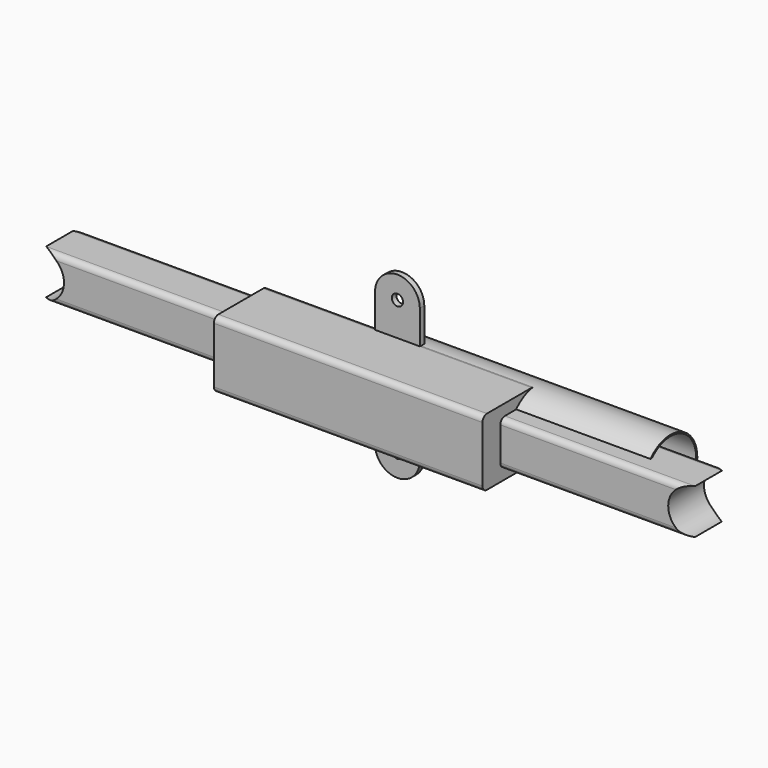
from build123d import *

# Parameters (mm, degrees)
F1_DEPTH    = 50.8
F2_R        = 6.35
F3_R        = 25.4
F3_R_2      = 22.225
F4_DEPTH    = 50.8
F6_DEPTH    = 50.8
F7_T1_DEPTH = 990.6
F8_R        = 6.35
F9_DEPTH    = 6.35
F10_R       = 22.225
F10_R_2     = 6.35
F11_DEPTH   = 50.8
F12_R       = 25.4
F12_R_2     = 6.35
F13_DEPTH   = 9.525
F14_R       = 38.1
F14_R_2     = 36.5506
F15_DEPTH   = 304.8
F16_R       = 6.35
F17_DEPTH   = 6.35
F18_W       = 304.8
F18_H       = 76.2
F19_DEPTH   = 76.2
F20_R       = 6.35


# Not quite as in the source:
# - a fillet or chamfer that OpenCascade refuses, or shapes differently, is made with other operations: its cross-section is extruded or revolved along the edge and cut away or added


with BuildPart() as f1:
    # F0 (on Front) → F1 (new body)
    with BuildSketch(Plane.XZ):
        with BuildLine():
            ThreePointArc((368.3, -25.4), (342.9, 0), (368.3, 25.4))
            Line((368.3, 25.4), (-368.3, 25.4))
            ThreePointArc((-368.3, 25.4), (-342.9, 0), (-368.3, -25.4))
            Line((-368.3, -25.4), (368.3, -25.4))
        make_face()
    extrude(amount=F1_DEPTH)

    # F2
    f2_edges = [f1.edges().sort_by_distance(p)[0] for p in [
        (0, -50.8, -25.4),
        (0, -50.8, 25.4),
        (0, 0, 25.4),
        (0, 0, -25.4),
    ]]
    fillet(f2_edges, radius=F2_R)


with BuildPart() as f4:
    # F3 (on Front) → F4 (new body)
    with BuildSketch(Plane.XZ):
        Circle(F3_R)
        Circle(F3_R_2, mode=Mode.SUBTRACT)
    extrude(amount=F4_DEPTH)


with BuildPart() as f6:
    # F5 (on Front) → F6 (new body)
    with BuildSketch(Plane.XZ):
        with BuildLine():
            ThreePointArc((368.3, -29.464), (338.836, 0), (368.3, 29.464))
            Line((368.3, 29.464), (-368.3, 29.464))
            ThreePointArc((-368.3, 29.464), (-338.836, 0), (-368.3, -29.464))
            Line((-368.3, -29.464), (368.3, -29.464))
        make_face()
    extrude(amount=F6_DEPTH)

    # F7: fillet of radius 50.8 on 4 edges, made by hand

    # F7_s2 → F7_t1 (cut)
    with BuildSketch(Plane.YZ.offset(-495.3)):
        with BuildLine():
            ThreePointArc((0, -29.464), (-35.9210244843, -14.5850244843), (-50.8, 21.336))
            Line((-50.8, 21.336), (-50.8, -29.464))
            Line((-50.8, -29.464), (0, -29.464))
        make_face()
        with BuildLine():
            ThreePointArc((0, 29.464), (-35.9210244843, 14.5850244843), (-50.8, -21.336))
            Line((-50.8, -21.336), (-50.8, 29.464))
            Line((-50.8, 29.464), (0, 29.464))
        make_face()
        with BuildLine():
            ThreePointArc((-50.8, -29.464), (-14.8789755157, -14.5850244843), (0, 21.336))
            Line((0, 21.336), (0, -29.464))
            Line((0, -29.464), (-50.8, -29.464))
        make_face()
        with BuildLine():
            ThreePointArc((-50.8, 29.464), (-14.8789755157, 14.5850244843), (0, -21.336))
            Line((0, -21.336), (0, 29.464))
            Line((0, 29.464), (-50.8, 29.464))
        make_face()
    extrude(amount=F7_T1_DEPTH, mode=Mode.SUBTRACT)


with BuildPart() as f9:
    # F8 (on Front) → F9 (new body)
    with BuildSketch(Plane.XZ):
        with BuildLine():
            Line((41.275, -50.8), (50.8, -50.8))
            Line((50.8, -50.8), (25.4, 25.4))
            ThreePointArc((25.4, 25.4), (0, 50.8), (-25.4, 25.4))
            Line((-25.4, 25.4), (-50.8, -50.8))
            Line((-50.8, -50.8), (-41.275, -50.8))
            ThreePointArc((-41.275, -50.8), (0, -9.525), (41.275, -50.8))
        make_face()
        with Locations((0, 25.4)):
            Circle(F8_R, mode=Mode.SUBTRACT)
    extrude(amount=F9_DEPTH)


with BuildPart() as f11:
    # F10 (on Front) → F11 (new body)
    with BuildSketch(Plane.XZ):
        Circle(F10_R)
        Circle(F10_R_2, mode=Mode.SUBTRACT)
    extrude(amount=F11_DEPTH)


with BuildPart() as f13:
    # F12 (on Front) → F13 (new body)
    with BuildSketch(Plane.XZ):
        Circle(F12_R)
        Circle(F12_R_2, mode=Mode.SUBTRACT)
    extrude(amount=F13_DEPTH)


with BuildPart() as f15:
    # F14 (on Right) → F15 (new body)
    with BuildSketch(Plane.YZ):
        Circle(F14_R)
        Circle(F14_R_2, mode=Mode.SUBTRACT)
    extrude(amount=F15_DEPTH)


with BuildPart() as f17:
    # F16 (on Front) → F17 (new body)
    with BuildSketch(Plane.XZ):
        with BuildLine():
            Line((25.4, -76.2), (25.4, 76.2))
            ThreePointArc((25.4, 76.2), (0, 101.6), (-25.4, 76.2))
            Line((-25.4, 76.2), (-25.4, 38.1))
            Line((-25.4, 38.1), (0, 38.1))
            Line((0, 38.1), (0, -38.1))
            Line((0, -38.1), (-25.4, -38.1))
            Line((-25.4, -38.1), (-25.4, -76.2))
            ThreePointArc((-25.4, -76.2), (0, -101.6), (25.4, -76.2))
        make_face()
        with Locations((0, -76.2)):
            Circle(F16_R, mode=Mode.SUBTRACT)
        with Locations((0, 76.2)):
            Circle(F16_R, mode=Mode.SUBTRACT)
    extrude(amount=F17_DEPTH)


with BuildPart() as f19:
    # F18 (on Front) → F19 (new body)
    with BuildSketch(Plane.XZ):
        Rectangle(F18_W, F18_H)
    extrude(amount=F19_DEPTH)

    # F20
    f20_edges = [f19.edges().sort_by_distance(p)[0] for p in [
        (0, -76.2, 38.1),
        (0, -76.2, -38.1),
        (0, 0, 38.1),
        (0, 0, -38.1),
    ]]
    fillet(f20_edges, radius=F20_R)


solid = Compound([f1.part, f4.part, f6.part, f9.part, f11.part, f13.part, f15.part, f17.part, f19.part])
